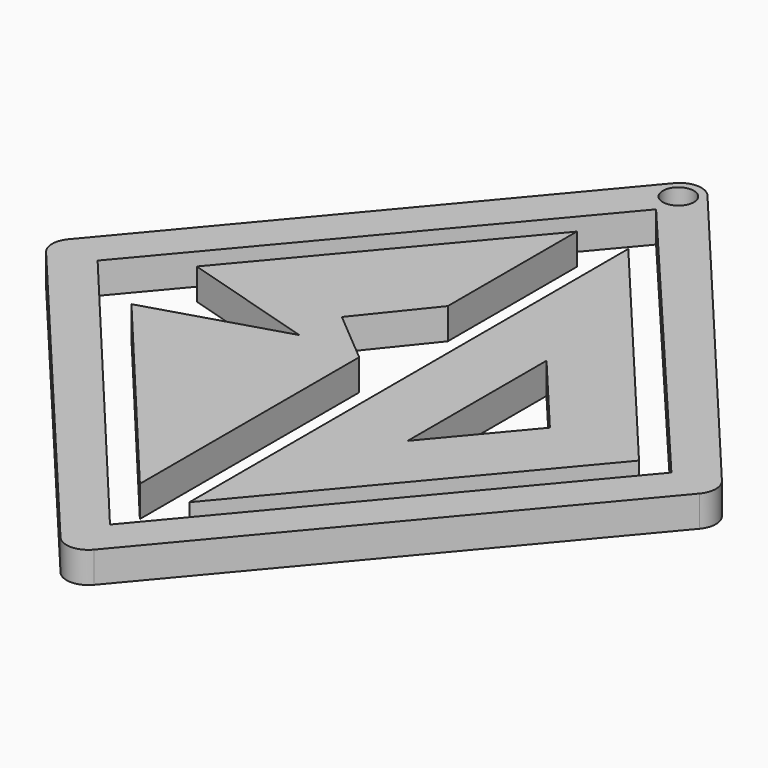
from build123d import *

# Parameters (mm, degrees)
F0_R     = 3.175
F1_DEPTH = 6.35


# Not quite as in the source:
# - a length typed as a fraction of an inch, garbled in the dataset ("3 / 203.2 mm" for 3/8 in), is restored


with BuildPart() as f1:
    # F0 (on Top) → F1 (new body)
    with BuildSketch(Plane.XY):
        with BuildLine():
            ThreePointArc((3.7735161073, 77.2181461795), (0.3684485576, 78.8059552545), (-3.036618992, 77.2181461795))
            Line((-3.036618992, 77.2181461795), (-66.5017581446, 1.5833385899))
            ThreePointArc((-66.5017581446, 1.5833385899), (-67.541690595, -1.2738523351), (-66.5017581446, -4.1310432602))
            Line((-66.5017581446, -4.1310432602), (-3.036618992, -79.7658508498))
            ThreePointArc((-3.036618992, -79.7658508498), (0.3684485576, -81.3536599247), (3.7735161073, -79.7658508498))
            Line((3.7735161073, -79.7658508498), (67.2386552599, -4.1310432602))
            ThreePointArc((67.2386552599, -4.1310432602), (68.2785877102, -1.2738523351), (67.2386552599, 1.5833385899))
            Line((67.2386552599, 1.5833385899), (3.7735161073, 77.2181461795))
        make_face()
        Polygon((0.3684485576, -71.3712848975), (-58.2422290914, -1.2738523351), (0.3684485576, 68.3287151025), (59.1871783672, -1.2738523351), align=None, mode=Mode.SUBTRACT)
        with Locations((0.3684485576, 74.0371476649)):
            Circle(F0_R, mode=Mode.SUBTRACT)
    extrude(amount=F1_DEPTH)


with BuildPart() as f1b:
    # F0 (on Top) → F1, piece 2 (new body)
    with BuildSketch(Plane.XY):
        Polygon((52.5557093374, -1.2738523351), (5.4484485576, 54.8663949365), (5.4484485576, -57.4140996067), align=None)
        Polygon((19.4184485576, -19.0318400569), (19.4184485576, 16.4841353867), (34.3191695055, -1.2738523351), align=None, mode=Mode.SUBTRACT)
    extrude(amount=F1_DEPTH)


with BuildPart() as f1c:
    # F0 (on Top) → F1, piece 3 (new body)
    with BuildSketch(Plane.XY):
        Polygon((-4.7115514424, 21.3924322091), (-4.7115514424, 54.4093134561), (-44.5979606519, 7.0425775949), (-16.9856430717, -1.2738523351), (-44.5979606519, -9.6726273153), (-4.7115514424, -57.3761344554), (-4.7115514424, -1.2738523351), (-15.5774667458, 7.87607823), align=None)
    extrude(amount=F1_DEPTH)


solid = Compound([f1.part, f1b.part, f1c.part])
